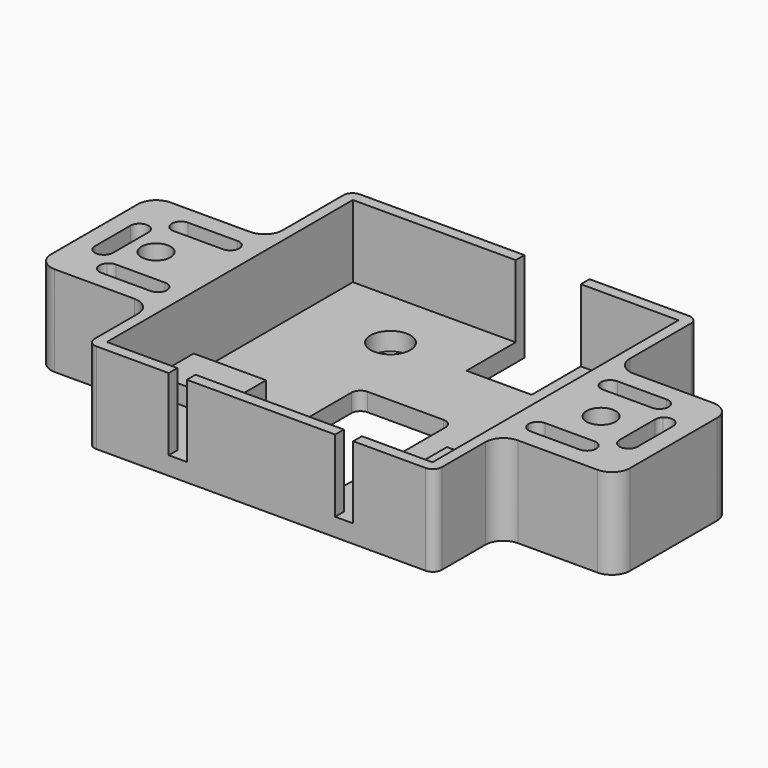
from build123d import *

# Parameters (mm, degrees)
F0_W      = 60.96
F0_H      = 57.785
F1_DEPTH  = 15.875
F2_W      = 57.15
F2_H      = 53.975
F3_DEPTH  = 12.7
F4_R      = 3.4925
F4_R_2    = 5.3975
F5_DEPTH  = 15.876
F6_W      = 12.7
F6_H      = 8.255
F7_DEPTH  = 3.175
F4_W      = 11.43
F4_H      = 12.7
F10_DEPTH = 25.4
F11_R     = 1.5875
F12_W     = 20.32
F12_H     = 25.4
F12_R     = 2.5527
F13_DEPTH = 15.875
F14_R     = 3.175
F15_R     = 1.58749
F16_W     = 3.175
F16_H     = 12.7
F17_DEPTH = 1.905


# Not quite as in the source:
# - a fillet or chamfer is up to 0.001 mm smaller than in the source, because OpenCascade refuses the exact size
# - a feature names something its author has since deleted; it is built from what else it names


with BuildPart() as f1:
    # F0 (on Top) → F1 (new body)
    with BuildSketch(Plane.XY):
        with Locations((30.48, 28.8925)):
            Rectangle(F0_W, F0_H)
    extrude(amount=F1_DEPTH)

    # F2 (on face) → F3 (cut)
    with BuildSketch(Plane.XY.offset(15.875)):
        with Locations((30.48, 28.8925)):
            Rectangle(F2_W, F2_H)
    extrude(amount=-F3_DEPTH, mode=Mode.SUBTRACT)

    # F4 (on face) → F5 (cut, through all)
    with BuildSketch(Plane(origin=(0, 0, 0), x_dir=(1, 0, 0), z_dir=(0, 0, -1))):
        with Locations((17.145, -45.085)):
            Circle(F4_R)
        with Locations((50.165, -45.085)):
            Circle(F4_R_2)
        with BuildLine():
            Line((37.1475, -5.08), (23.8125, -5.08))
            ThreePointArc((23.8125, -5.08), (22.6899679849, -5.5449679849), (22.225, -6.6675))
            Line((22.225, -6.6675), (22.225, -30.1625))
            ThreePointArc((22.225, -30.1625), (22.6899679849, -31.2850320151), (23.8125, -31.75))
            Line((23.8125, -31.75), (37.1475, -31.75))
            ThreePointArc((37.1475, -31.75), (38.2700320151, -31.2850320151), (38.735, -30.1625))
            Line((38.735, -30.1625), (38.735, -6.6675))
            ThreePointArc((38.735, -6.6675), (38.2700320151, -5.5449679849), (37.1475, -5.08))
        make_face()
    extrude(amount=-F5_DEPTH, mode=Mode.SUBTRACT)

    # F6 (on face) → F7 (join)
    with BuildSketch(Plane.XY.offset(3.175)):
        with Locations((8.255, 16.8275)):
            Rectangle(F6_W, F6_H)
        with Locations((52.705, 16.8275)):
            Rectangle(F6_W, F6_H)
    extrude(amount=F7_DEPTH)

    # F4 (on face) → F10 (cut)
    with BuildSketch(Plane(origin=(0, 0, 0), x_dir=(1, 0, 0), z_dir=(0, 0, -1))):
        with Locations((36.195, -51.435)):
            Rectangle(F4_W, F4_H)
    extrude(amount=-F10_DEPTH, mode=Mode.SUBTRACT)

    # F11
    f11_edges = [f1.edges().sort_by_distance(p)[0] for p in [
        (0, 57.785, 7.9375),
        (0, 0, 7.9375),
        (60.96, 57.785, 7.9375),
        (60.96, 0, 7.9375),
    ]]
    fillet(f11_edges, radius=F11_R)

    # F12 (on Top) → F13 (join, through all)
    with BuildSketch(Plane.XY):
        with Locations((-10.16, 26.9875)):
            Rectangle(F12_W, F12_H)
        with Locations((-9.525, 26.9875)):
            Circle(F12_R, mode=Mode.SUBTRACT)
        Polygon((-12.1739487758, 20.6375), (-1.27, 20.6375), (-1.27, 17.4625), (-15.3489487758, 17.4625), (-17.145, 17.4625), (-17.145, 19.2585512242), (-17.145, 34.7164487758), (-17.145, 36.5125), (-15.3489487758, 36.5125), (-1.27, 36.5125), (-1.27, 33.3375), (-12.1739487758, 33.3375), (-13.97, 33.3375), (-13.97, 31.5414487758), (-13.97, 22.4335512242), (-13.97, 20.6375), align=None, mode=Mode.SUBTRACT)
        with Locations((71.12, 26.9875)):
            Rectangle(F12_W, F12_H)
        with Locations((68.58, 26.9875)):
            Circle(F12_R, mode=Mode.SUBTRACT)
        Polygon((76.3089487758, 17.4625), (62.23, 17.4625), (62.23, 20.6375), (73.1339487758, 20.6375), (74.93, 20.6375), (74.93, 22.4335512242), (74.93, 31.5414487758), (74.93, 33.3375), (73.1339487758, 33.3375), (62.23, 33.3375), (62.23, 36.5125), (76.3089487758, 36.5125), (78.105, 36.5125), (78.105, 34.7164487758), (78.105, 19.2585512242), (78.105, 17.4625), align=None, mode=Mode.SUBTRACT)
        Polygon((73.1339487758, 20.6375), (76.3089487758, 17.4625), (78.105, 17.4625), (78.105, 19.2585512242), (74.93, 22.4335512242), (74.93, 20.6375), align=None)
        Polygon((74.93, 31.5414487758), (78.105, 34.7164487758), (78.105, 36.5125), (76.3089487758, 36.5125), (73.1339487758, 33.3375), (74.93, 33.3375), align=None)
        Polygon((-17.145, 34.7164487758), (-13.97, 31.5414487758), (-13.97, 33.3375), (-12.1739487758, 33.3375), (-15.3489487758, 36.5125), (-17.145, 36.5125), align=None)
        Polygon((-15.3489487758, 17.4625), (-12.1739487758, 20.6375), (-13.97, 20.6375), (-13.97, 22.4335512242), (-17.145, 19.2585512242), (-17.145, 17.4625), align=None)
    extrude(amount=F13_DEPTH)

    # F14
    f14_edges = [f1.edges().sort_by_distance(p)[0] for p in [
        (-20.32, 14.2875, 7.9375),
        (0, 14.2875, 7.9375),
        (-20.32, 39.6875, 7.9375),
        (0, 39.6875, 7.9375),
        (60.96, 14.2875, 7.9375),
        (81.28, 14.2875, 7.9375),
        (81.28, 39.6875, 7.9375),
        (60.96, 39.6875, 7.9375),
    ]]
    fillet(f14_edges, radius=F14_R)

    # F15 (radius 1.5875 in the source; OpenCascade refuses exactly that, so slightly less here)
    f15_edges = [f1.edges().sort_by_distance(p)[0] for p in [
        (62.23, 17.4625, 7.9375),
        (62.23, 20.6375, 7.9375),
        (62.23, 33.3375, 7.9375),
        (62.23, 36.5125, 7.9375),
        (76.308949, 17.4625, 7.9375),
        (78.105, 19.258551, 7.9375),
        (78.105, 34.716449, 7.9375),
        (74.93, 31.541449, 7.9375),
        (74.93, 22.433551, 7.9375),
        (73.133949, 20.6375, 7.9375),
        (73.133949, 33.3375, 7.9375),
        (76.308949, 36.5125, 7.9375),
        (-1.27, 33.3375, 7.9375),
        (-1.27, 36.5125, 7.9375),
        (-15.348949, 36.5125, 7.9375),
        (-12.173949, 33.3375, 7.9375),
        (-15.348949, 17.4625, 7.9375),
        (-12.173949, 20.6375, 7.9375),
        (-1.27, 17.4625, 7.9375),
        (-1.27, 20.6375, 7.9375),
        (-17.145, 19.258551, 7.9375),
        (-13.97, 22.433551, 7.9375),
        (-17.145, 34.716449, 7.9375),
        (-13.97, 31.541449, 7.9375),
    ]]
    fillet(f15_edges, radius=F15_R)

    # F16 (on face) → F17 (cut, through all)
    with BuildSketch(Plane.XZ):
        with Locations((15.875, 9.525)):
            Rectangle(F16_W, F16_H)
        with Locations((45.085, 9.525)):
            Rectangle(F16_W, F16_H)
    extrude(amount=-F17_DEPTH, mode=Mode.SUBTRACT)


solid = f1.part
